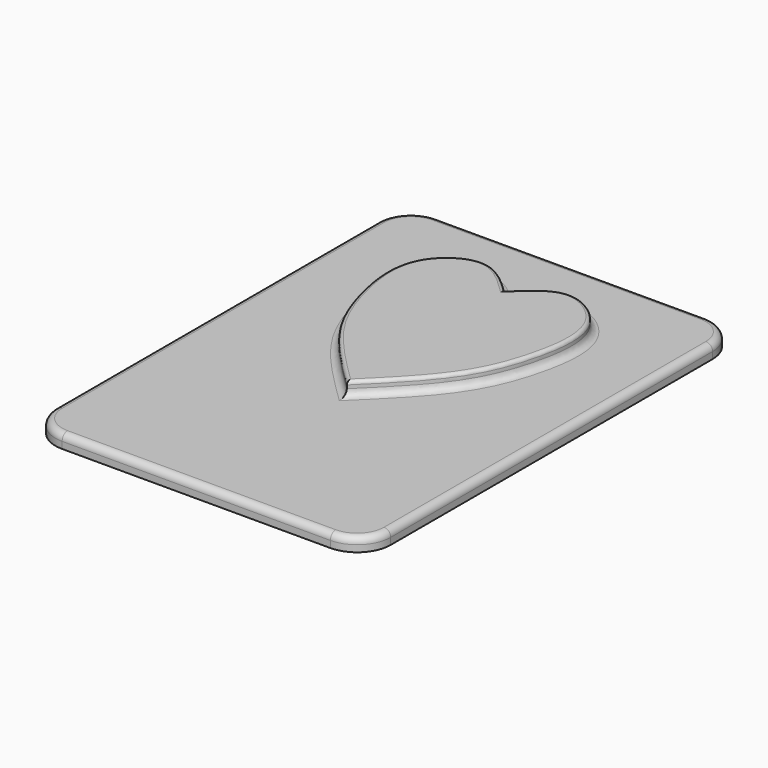
from build123d import *

# Parameters (mm, degrees)
F1_DEPTH = 5.08
F3_DEPTH = 5.08
F4_R     = 1.27
F5_R     = 2.54


with BuildPart() as f1:
    # F0 (on Top) → F1 (new body)
    with BuildSketch(Plane.XY):
        with BuildLine():
            ThreePointArc((0, 12.7), (3.7197438789, 3.7197438789), (12.7, 0))
            Line((12.7, 0), (114.3, 0))
            ThreePointArc((114.3, 0), (123.2802561211, 3.7197438789), (127, 12.7))
            Line((127, 12.7), (127, 165.1))
            ThreePointArc((127, 165.1), (123.2802561211, 174.0802561211), (114.3, 177.8))
            Line((114.3, 177.8), (12.7, 177.8))
            ThreePointArc((12.7, 177.8), (3.7197438789, 174.0802561211), (0, 165.1))
            Line((0, 165.1), (0, 12.7))
        make_face()
    extrude(amount=F1_DEPTH)

    # F2 (on face) → F3 (join)
    with BuildSketch(Plane.XY.offset(5.08)):
        with BuildLine():
            add(Edge.make_bspline(
                [(63.5, 145.9377408028), (68.6348735634, 150.9255986286), (78.941516072, 160.9371533165), (100.50869854, 146.40526225), (97.4644485377, 120.6257253689), (90.046447698, 100.4861086213), (77.8216215421, 85.3028694811), (68.3139614105, 76.0008236819), (63.5, 71.2909698486)],
                knots=[0, 0, 0, 0, 0.1610044671, 0.3231657926, 0.5037663014, 0.6750092725, 0.8354492273, 1, 1, 1, 1], degree=3))
            add(Edge.make_bspline(
                [(63.5, 145.9377408028), (58.3651264366, 150.9255986286), (48.058483928, 160.9371533165), (26.49130146, 146.40526225), (29.5355514623, 120.6257253689), (36.953552302, 100.4861086213), (49.1783784579, 85.3028694811), (58.6860385895, 76.0008236819), (63.5, 71.2909698486)],
                knots=[0, 0, 0, 0, 0.1610044671, 0.3231657926, 0.5037663014, 0.6750092725, 0.8354492273, 1, 1, 1, 1], degree=3))
        make_face()
    extrude(amount=F3_DEPTH)

    # F4
    f4_edges = [f1.edges().sort_by_distance(p)[0] for p in [
        (97.022157, 122.999837, 10.16),
        (29.977843, 122.999837, 10.16),
    ]]
    fillet(f4_edges, radius=F4_R)

    # F5
    f5_edges = [f1.edges().sort_by_distance(p)[0] for p in [
        (0, 88.9, 5.08),
        (3.719744, 174.080256, 5.08),
        (3.719744, 3.719744, 5.08),
        (63.5, 177.8, 5.08),
        (63.5, 0, 5.08),
        (123.280256, 174.080256, 5.08),
        (123.280256, 3.719744, 5.08),
        (127, 88.9, 5.08),
        (29.977843, 122.999837, 5.08),
        (97.022157, 122.999837, 5.08),
    ]]
    fillet(f5_edges, radius=F5_R)


solid = f1.part
